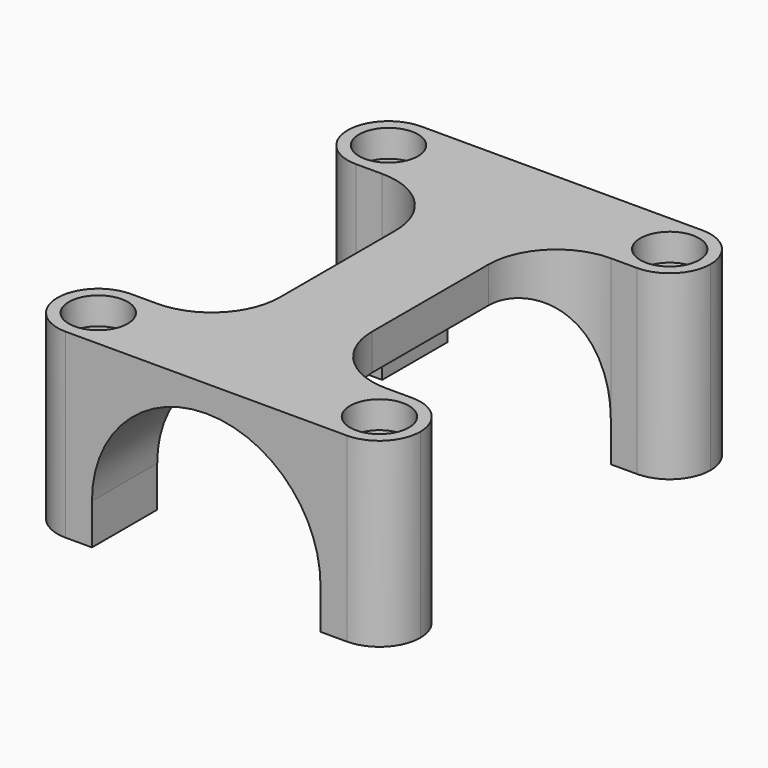
from build123d import *

# Parameters (mm, degrees)
F1_DEPTH       = 49
F3_D           = 3.3
F3_DEPTH       = 30
F3_CBORE_D     = 6.5
F3_CBORE_DEPTH = 3
F3_TIP         = 0.9914200214
F5_DEPTH       = 25
F6_R           = 4.49999


# Not quite as in the source:
# - a fillet or chamfer is up to 0.001 mm smaller than in the source, because OpenCascade refuses the exact size


with BuildPart() as f1:
    # F0 (on Front) → F1 (new body)
    with BuildSketch(Plane.XZ):
        with BuildLine():
            Line((0, 20), (0, 0))
            Line((0, 0), (7.4, 0))
            Line((7.4, 0), (7.4, 4.5))
            ThreePointArc((7.4, 4.5), (20, 17.1), (32.6, 4.5))
            Line((32.6, 4.5), (32.6, 0))
            Line((32.6, 0), (40, 0))
            Line((40, 0), (40, 20))
            Line((40, 20), (0, 20))
        make_face()
    extrude(amount=F1_DEPTH)

    # F3
    with Locations(Plane.XY.offset(20)):
        with Locations((4.5, -4.5), (4.5, -44.5), (35.5, -44.5), (35.5, -4.5)):
            CounterBoreHole(F3_D / 2, F3_CBORE_D / 2, F3_CBORE_DEPTH, depth=F3_DEPTH)
            with Locations((0, 0, -(F3_DEPTH + F3_TIP / 2))):  # 118° drill point
                Cone(0, F3_D / 2, F3_TIP, mode=Mode.SUBTRACT)

    # F4 (on face) → F5 (cut)
    with BuildSketch(Plane.XY.offset(20)):
        with BuildLine():
            Line((14.9, -32.5), (14.9, -16.5))
            ThreePointArc((14.9, -16.5), (12.7033008589, -11.1966991411), (7.4, -9))
            Line((7.4, -9), (-0.1, -9))
            Line((-0.1, -9), (-0.1, -40))
            Line((-0.1, -40), (7.4, -40))
            ThreePointArc((7.4, -40), (12.7033008589, -37.8033008589), (14.9, -32.5))
        make_face()
        with BuildLine():
            ThreePointArc((32.6, -9), (27.2966991411, -11.1966991411), (25.1, -16.5))
            Line((25.1, -16.5), (25.1, -32.5))
            ThreePointArc((25.1, -32.5), (27.2966991411, -37.8033008589), (32.6, -40))
            Line((32.6, -40), (40.1, -40))
            Line((40.1, -40), (40.1, -9))
            Line((40.1, -9), (32.6, -9))
        make_face()
    extrude(amount=-F5_DEPTH, mode=Mode.SUBTRACT)

    # F6 (radius 4.5 in the source; OpenCascade refuses exactly that, so slightly less here)
    f6_edges = [f1.edges().sort_by_distance(p)[0] for p in [
        (40, -49, 10),
        (0, -49, 10),
        (40, 0, 10),
        (0, 0, 10),
        (40, -9, 10),
        (40, -40, 10),
        (0, -40, 10),
        (0, -9, 10),
    ]]
    fillet(f6_edges, radius=F6_R)


solid = f1.part
